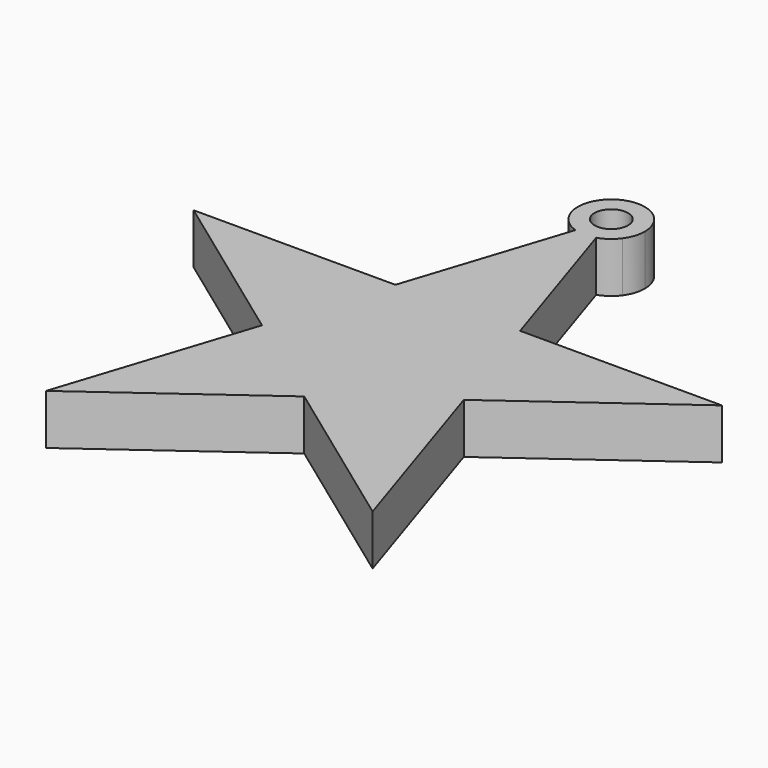
from build123d import *

# Parameters (mm, degrees)
F1_DEPTH = 3


# Not quite as in the source:
# - a feature names something its author has since deleted; it is built from what else it names


with BuildPart() as f1:
    # F0 (on Top) → F1 (new body)
    with BuildSketch(Plane.XY):
        with BuildLine():
            ThreePointArc((0.6180339887, 14.6814791024), (0, 14.583592135), (-0.6180339887, 14.6814791024))
            Line((-0.6180339887, 14.6814791024), (-3.7232484104, 5.1246117975))
            Line((-3.7232484104, 5.1246117975), (-15.7719333636, 5.1246117975))
            Line((-15.7719333636, 5.1246117975), (-6.0243424766, -1.9574275275))
            Line((-6.0243424766, -1.9574275275), (-9.747590887, -13.416407865))
            Line((-9.747590887, -13.416407865), (0, -6.33436854))
            Line((0, -6.33436854), (9.747590887, -13.416407865))
            Line((9.747590887, -13.416407865), (6.0243424766, -1.9574275275))
            Line((6.0243424766, -1.9574275275), (15.7719333636, 5.1246117975))
            Line((15.7719333636, 5.1246117975), (3.7232484104, 5.1246117975))
            Line((3.7232484104, 5.1246117975), (0.6180339887, 14.6814791024))
        make_face()
        with BuildLine():
            ThreePointArc((0.3090169944, 15.6325356187), (0, 15.583592135), (-0.3090169944, 15.6325356187))
            Line((-0.3090169944, 15.6325356187), (-0.6180339887, 14.6814791024))
            ThreePointArc((-0.6180339887, 14.6814791024), (0, 14.583592135), (0.6180339887, 14.6814791024))
            Line((0.6180339887, 14.6814791024), (0.3090169944, 15.6325356187))
        make_face()
        with BuildLine():
            Line((1.6180339887, 15.4080216304), (0.8090169944, 15.9958068827))
            ThreePointArc((0.8090169944, 15.9958068827), (0.5877852523, 15.7745751406), (0.3090169944, 15.6325356187))
            Line((0.3090169944, 15.6325356187), (0.6180339887, 14.6814791024))
            ThreePointArc((0.6180339887, 14.6814791024), (1.1755705046, 14.9655581463), (1.6180339887, 15.4080216304))
        make_face()
        with BuildLine():
            ThreePointArc((1, 16.583592135), (0.9510565163, 16.2745751406), (0.8090169944, 15.9958068827))
            Line((0.8090169944, 15.9958068827), (1.6180339887, 15.4080216304))
            ThreePointArc((1.6180339887, 15.4080216304), (1.9021130326, 15.9655581463), (2, 16.583592135))
            ThreePointArc((2, 16.583592135), (-0.6180339887, 18.4857051676), (-1.6180339887, 15.4080216304))
            Line((-1.6180339887, 15.4080216304), (-0.8090169944, 15.9958068827))
            ThreePointArc((-0.8090169944, 15.9958068827), (-0.3090169944, 17.5346486513), (1, 16.583592135))
        make_face()
        with BuildLine():
            ThreePointArc((-0.3090169944, 15.6325356187), (-0.5877852523, 15.7745751406), (-0.8090169944, 15.9958068827))
            Line((-0.8090169944, 15.9958068827), (-1.6180339887, 15.4080216304))
            ThreePointArc((-1.6180339887, 15.4080216304), (-1.1755705046, 14.9655581463), (-0.6180339887, 14.6814791024))
            Line((-0.6180339887, 14.6814791024), (-0.3090169944, 15.6325356187))
        make_face()
    extrude(amount=F1_DEPTH)


solid = f1.part
